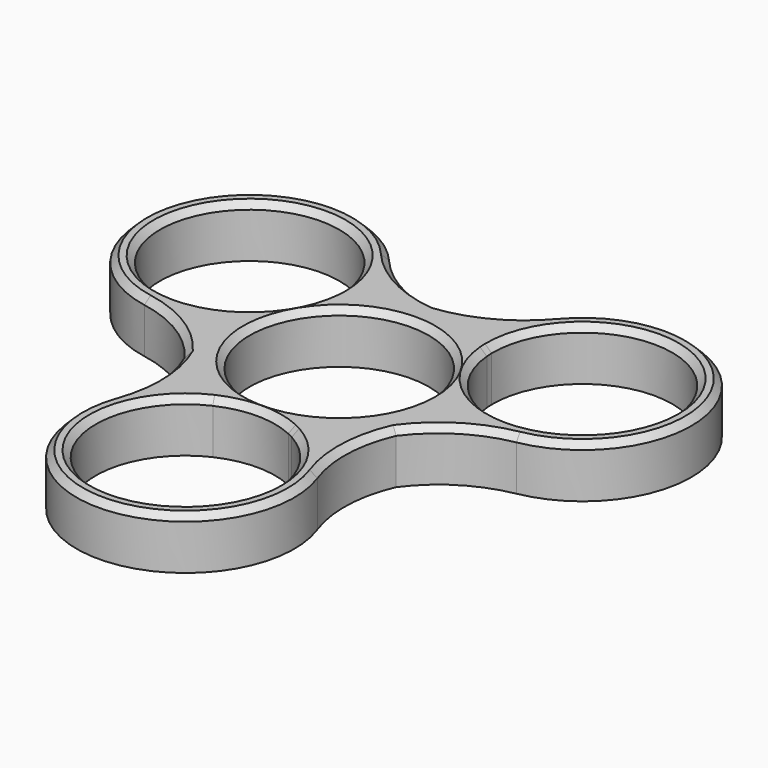
from build123d import *

# Parameters (mm, degrees)
F0_R        = 14
F1_DEPTH    = 8.05
F2_T1_DEPTH = 8.05
F3_SIZE     = 0.99999


# Not quite as in the source:
# - a fillet or chamfer that OpenCascade refuses, or shapes differently, is made with other operations: its cross-section is extruded or revolved along the edge and cut away or added
# - a fillet or chamfer is up to 0.001 mm smaller than in the source, because OpenCascade refuses the exact size


with BuildPart() as f1:
    # F0 (on Top) → F1 (new body)
    with BuildSketch(Plane.XY):
        with BuildLine():
            ThreePointArc((-18.9934809997, -0.4976741041), (-16.4544826719, -9.5), (-9.9277389168, -16.2))
            ThreePointArc((-9.9277389168, -16.2), (0, -47), (9.9277389168, -16.2))
            ThreePointArc((9.9277389168, -16.2), (16.4544826719, -9.5), (18.9934809997, -0.4976741041))
            ThreePointArc((18.9934809997, -0.4976741041), (40.7031939779, 23.5), (9.0657420829, 16.6976741041))
            ThreePointArc((9.0657420829, 16.6976741041), (0, 19), (-9.0657420829, 16.6976741041))
            ThreePointArc((-9.0657420829, 16.6976741041), (-40.7031939779, 23.5), (-18.9934809997, -0.4976741041))
        make_face()
        with BuildLine():
            ThreePointArc((5.9, -17.3039376183), (6.3427828622, -17.5192506009), (6.7777208559, -17.75))
            ThreePointArc((6.7777208559, -17.75), (12.0600184905, -22.8897289778), (14, -30))
            ThreePointArc((14, -30), (-7.5299402388, -41.8025420991), (-5.9, -17.3039376183))
            ThreePointArc((-5.9, -17.3039376183), (0, -16), (5.9, -17.3039376183))
        make_face(mode=Mode.SUBTRACT)
        with BuildLine():
            ThreePointArc((-17.9356495629, 3.5424189268), (-38.4031526988, 21.4563311676), (-11.9807621135, 15))
            ThreePointArc((-11.9807621135, 15), (-11.9944907071, 14.3801515137), (-12.0356495629, 13.7615186915))
            ThreePointArc((-12.0356495629, 13.7615186915), (-13.8564064606, 8), (-17.9356495629, 3.5424189268))
        make_face(mode=Mode.SUBTRACT)
        Circle(F0_R, mode=Mode.SUBTRACT)
        with BuildLine():
            ThreePointArc((11.9830904892, 14.7446784409), (25.8530960258, 28.999417894), (39.9807621135, 15))
            ThreePointArc((39.9807621135, 15), (32.4370932811, 2.5776094147), (17.9356495629, 3.5424189268))
            ThreePointArc((17.9356495629, 3.5424189268), (13.8564064606, 8), (12.0356495629, 13.7615186915))
            ThreePointArc((12.0356495629, 13.7615186915), (12.0007246446, 14.2526363898), (11.9830904892, 14.7446784409))
        make_face(mode=Mode.SUBTRACT)
    extrude(amount=F1_DEPTH)

    # F2: fillet of radius 20 on 6 edges, made by hand

    # F2_s2 → F2_t1 (join)
    with BuildSketch(Plane.XY):
        with BuildLine():
            ThreePointArc((-15.8833011878, -10.4269239653), (-21.5600561339, -4.7274127209), (-29.0232123622, -1.725534266))
            ThreePointArc((-29.0232123622, -1.725534266), (-23.9150097608, -1.8740234448), (-18.9934809997, -0.4976741041))
            ThreePointArc((-18.9934809997, -0.4976741041), (-18.1313260585, -5.6793499065), (-15.8833011878, -10.4269239653))
        make_face()
        with BuildLine():
            ThreePointArc((-16.9716316312, -8.5418803419), (-14.8740875774, -16.3078499586), (-16.0059626906, -24.2720720721))
            ThreePointArc((-16.0059626906, -24.2720720721), (-13.5804567909, -19.7739942621), (-9.9277389168, -16.2))
            ThreePointArc((-9.9277389168, -16.2), (-13.9841243252, -12.8625140177), (-16.9716316312, -8.5418803419))
        make_face()
        with BuildLine():
            ThreePointArc((-1.0883304434, 18.9688043072), (6.6859685565, 21.0352626795), (13.0172496716, 25.9976063381))
            ThreePointArc((13.0172496716, 25.9976063381), (10.3345529699, 21.648017707), (9.0657420829, 16.6976741041))
            ThreePointArc((9.0657420829, 16.6976741041), (4.1472017333, 18.5418639242), (-1.0883304434, 18.9688043072))
        make_face()
        with BuildLine():
            ThreePointArc((1.0883304434, 18.9688043072), (-6.6859685565, 21.0352626795), (-13.0172496716, 25.9976063381))
            ThreePointArc((-13.0172496716, 25.9976063381), (-10.3345529699, 21.648017707), (-9.0657420829, 16.6976741041))
            ThreePointArc((-9.0657420829, 16.6976741041), (-4.1472017333, 18.5418639242), (1.0883304434, 18.9688043072))
        make_face()
        with BuildLine():
            ThreePointArc((29.0232123622, -1.725534266), (21.5600561339, -4.7274127209), (15.8833011878, -10.4269239653))
            ThreePointArc((15.8833011878, -10.4269239653), (18.1313260585, -5.6793499065), (18.9934809997, -0.4976741041))
            ThreePointArc((18.9934809997, -0.4976741041), (23.9150097608, -1.8740234448), (29.0232123622, -1.725534266))
        make_face()
        with BuildLine():
            ThreePointArc((16.9716316312, -8.5418803419), (14.8740875774, -16.3078499586), (16.0059626906, -24.2720720721))
            ThreePointArc((16.0059626906, -24.2720720721), (13.5804567909, -19.7739942621), (9.9277389168, -16.2))
            ThreePointArc((9.9277389168, -16.2), (13.9841243252, -12.8625140177), (16.9716316312, -8.5418803419))
        make_face()
    extrude(amount=F2_T1_DEPTH)

    # F3 (size 1 in the source; OpenCascade refuses exactly that, so slightly less here)
    f3_edges = [f1.edges().sort_by_distance(p)[0] for p in [
        (0, -47, 8.05),
        (14.848068, -16.8534, 8.05),
        (22.019507, -4.432104, 8.05),
        (40.703194, 23.5, 8.05),
        (7.171439, 21.285504, 8.05),
        (-7.171439, 21.285504, 8.05),
        (-40.703194, 23.5, 8.05),
        (-22.019507, -4.432104, 8.05),
        (-14.848068, -16.8534, 8.05),
        (5.9, -42.696062, 8.05),
        (-39.980762, 15, 8.05),
        (-14, 0, 8.05),
        (11.980762, 15, 8.05),
    ]]
    chamfer(f3_edges, length=F3_SIZE)


solid = f1.part
